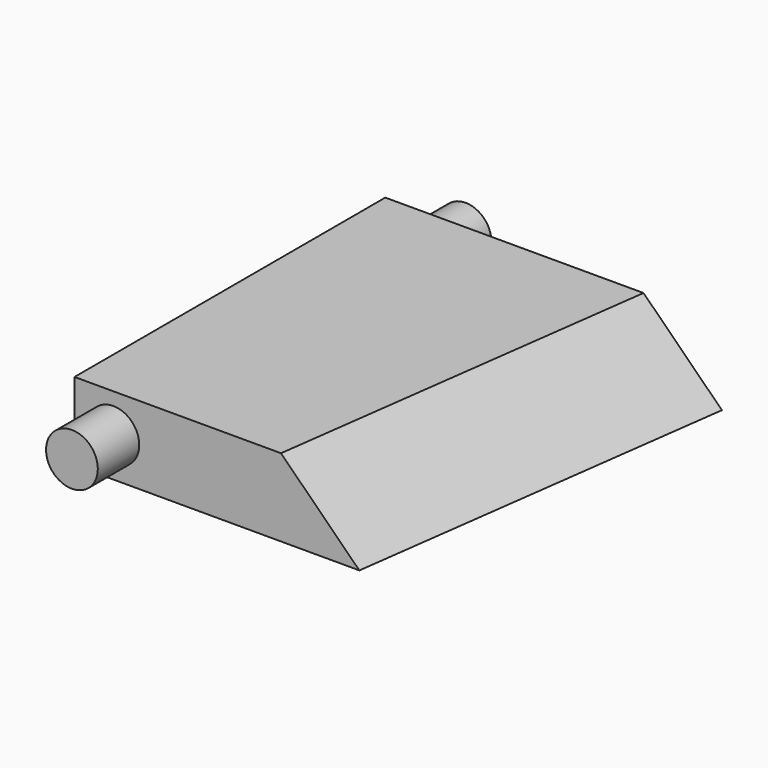
from build123d import *

# Parameters (mm, degrees)
F1_DEPTH = 3
F2_SIZE2 = 2.99999
F2_SIZE  = 2.99999
F3_R     = 1
F4_DEPTH = 2
F5_R     = 1
F6_DEPTH = 2


# Not quite as in the source:
# - a fillet or chamfer is up to 0.001 mm smaller than in the source, because OpenCascade refuses the exact size


with BuildPart() as f1:
    # F0 (on Top) → F1 (new body)
    with BuildSketch(Plane.XY):
        Polygon((11, 3), (11, 0), (22, 0), (24, 15), (11, 15), (11, 12), align=None)
    extrude(amount=F1_DEPTH)

    # F2 (size 3 and 3 in the source; OpenCascade refuses exactly that, so slightly less here)
    f2_edges = [f1.edges().sort_by_distance(p)[0] for p in [
        (23, 7.5, 3),
    ]]
    chamfer(f2_edges, length=F2_SIZE, length2=F2_SIZE2)

    # F3 (on face) → F4 (join)
    with BuildSketch(Plane.XZ):
        with Locations((12.5, 1.5)):
            Circle(F3_R)
    extrude(amount=F4_DEPTH)

    # F5 (on face) → F6 (join)
    with BuildSketch(Plane(origin=(0, 15, 0), x_dir=(-1, 0, 0), z_dir=(0, 1, 0))):
        with Locations((-12.5, 1.5)):
            Circle(F5_R)
    extrude(amount=F6_DEPTH)


solid = f1.part
